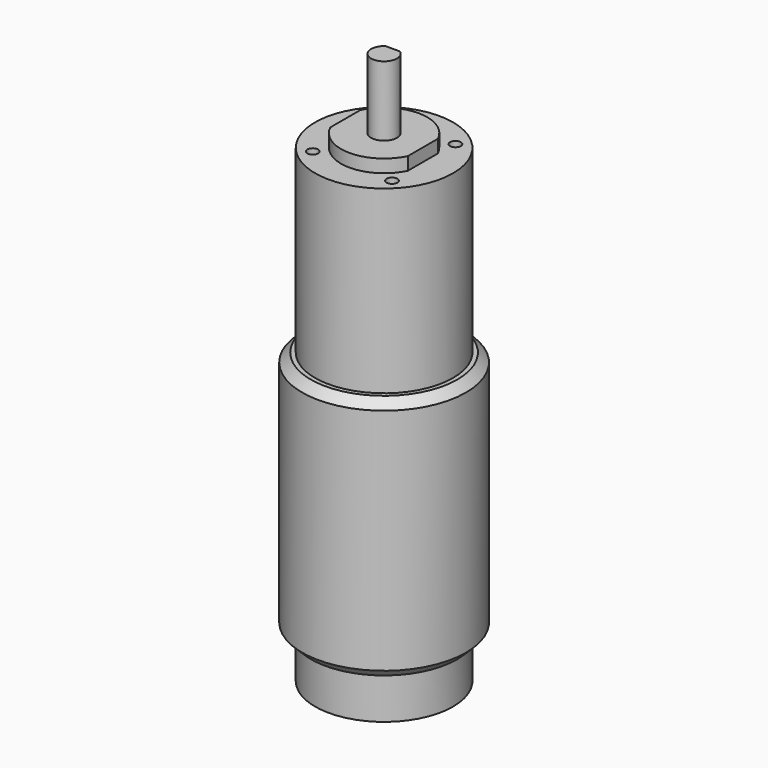
from build123d import *

# Parameters (mm, degrees)
F0_R      = 19
F1_DEPTH  = 57.1
F2_R      = 16
F3_DEPTH  = 41.8
F4_R      = 16
F5_DEPTH  = 10
F7_DEPTH  = 3
F8_R      = 3
F9_DEPTH  = 16.2
F10_W     = 3.3166247904
F10_H     = 0.5
F11_DEPTH = 12
F12_SIZE  = 2
F14_D     = 2.5
F14_DEPTH = 13.5
F14_TIP   = 0.7510757738


with BuildPart() as f1:
    # F0 (on Top) → F1 (new body)
    with BuildSketch(Plane.XY):
        Circle(F0_R)
    extrude(amount=-F1_DEPTH)

    # F2 (on face) → F3 (join)
    with BuildSketch(Plane.XY):
        Circle(F2_R)
    extrude(amount=F3_DEPTH)

    # F4 (on face) → F5 (join)
    with BuildSketch(Plane(origin=(0, 0, -57.1), x_dir=(1, 0, 0), z_dir=(0, 0, -1))):
        Circle(F4_R)
    extrude(amount=F5_DEPTH)

    # F6 (on face) → F7 (join)
    with BuildSketch(Plane.XY.offset(41.8)):
        with BuildLine():
            ThreePointArc((9, 4.3588989435), (0, 10), (-9, 4.3588989435))
            Line((-9, 4.3588989435), (-9, -4.3588989435))
            ThreePointArc((-9, -4.3588989435), (0, -10), (9, -4.3588989435))
            Line((9, -4.3588989435), (9, 4.3588989435))
        make_face()
    extrude(amount=F7_DEPTH)

    # F8 (on face) → F9 (join)
    with BuildSketch(Plane.XY.offset(44.8)):
        Circle(F8_R)
    extrude(amount=F9_DEPTH)

    # F10 (on face) → F11 (cut)
    with BuildSketch(Plane.XY.offset(61)):
        with Locations((0, 2.75)):
            Rectangle(F10_W, F10_H)
    extrude(amount=-F11_DEPTH, mode=Mode.SUBTRACT)

    # F12
    f12_edges = [f1.edges().sort_by_distance(p)[0] for p in [
        (-19, 0, -57.1),
        (-19, 0, 0),
    ]]
    chamfer(f12_edges, length=F12_SIZE)

    # F14
    with Locations(Plane.XY.offset(41.8)):
        with Locations((-9.1923881554, 9.1923881554), (9.1923881554, 9.1923881554), (9.1923881554, -9.1923881554), (-9.1923881554, -9.1923881554)):
            Hole(F14_D / 2, depth=F14_DEPTH)
            with Locations((0, 0, -(F14_DEPTH + F14_TIP / 2))):  # 118° drill point
                Cone(0, F14_D / 2, F14_TIP, mode=Mode.SUBTRACT)


solid = f1.part
